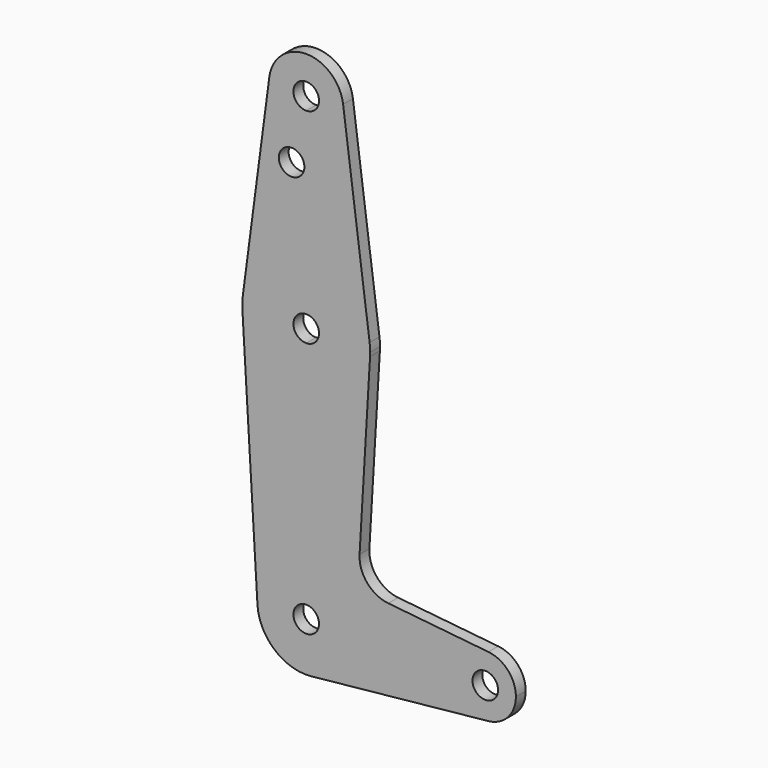
from build123d import *

# Parameters (mm, degrees)
F0_R     = 3.175
F1_DEPTH = 3.048


with BuildPart() as f1:
    # F0 (on Front) → F1 (new body)
    with BuildSketch(Plane.XZ):
        with BuildLine():
            Line((12.1285329959, 0), (3.175, 0))
            ThreePointArc((3.175, 0), (-2.2450640303, -2.2450640303), (0, 3.175))
            Line((0, 3.175), (0, 12.1285329959))
            ThreePointArc((0, 12.1285329959), (-8.8255371973, 8.3193272451), (-12.1074052539, -0.7155771445))
            ThreePointArc((-12.1074052539, -0.7155771445), (-7.858618829, -9.2381503956), (1.2349249899, -12.0654992811))
            ThreePointArc((1.2349249899, -12.0654992811), (9.002198096, -8.1278374782), (12.1285329959, 0))
        make_face()
        with BuildLine():
            ThreePointArc((0, 12.1285329959), (8.5761679272, 8.5761679272), (12.1285329959, 0))
            Line((12.1285329959, 0), (36.8473577956, 0))
            ThreePointArc((36.8473577956, 0), (39.3551513268, 5.6429323481), (45.2240996253, 7.5631301892))
            Line((45.2240996253, 7.5631301892), (20.3690705941, 10.1070859559))
            ThreePointArc((20.3690705941, 10.1070859559), (15.1229915635, 12.8646775774), (13.2422076318, 18.4850253022))
            Line((13.2422076318, 18.4850253022), (15.8473459627, 62.563383249))
            ThreePointArc((15.8473459627, 62.563383249), (10.8891421627, 51.9482811685), (0, 47.625))
            Line((0, 47.625), (0, 12.1285329959))
        make_face()
        with BuildLine():
            Line((36.8473577956, 0), (12.1285329959, 0))
            ThreePointArc((12.1285329959, 0), (9.002198096, -8.1278374782), (1.2349249899, -12.0654992811))
            Line((1.2349249899, -12.0654992811), (45.2240996253, -7.5631301892))
            ThreePointArc((45.2240996253, -7.5631301892), (39.3551513268, -5.6429323481), (36.8473577956, 0))
        make_face()
        with BuildLine():
            ThreePointArc((-12.1074052539, -0.7155771445), (-8.8255371973, 8.3193272451), (0, 12.1285329959))
            Line((0, 12.1285329959), (0, 47.625))
            ThreePointArc((0, 47.625), (-10.8891421627, 51.9482811685), (-15.8473459627, 62.563383249))
            Line((-15.8473459627, 62.563383249), (-12.1074052539, -0.7155771445))
        make_face()
        with BuildLine():
            ThreePointArc((45.2240996253, 7.5631301892), (39.3551513268, 5.6429323481), (36.8473577956, 0))
            ThreePointArc((36.8473577956, 0), (39.3551513268, -5.6429323481), (45.2240996253, -7.5631301892))
            ThreePointArc((45.2240996253, -7.5631301892), (50.0929323481, -5.0948486732), (52.0526422044, 0))
            ThreePointArc((52.0526422044, 0), (50.0929323481, 5.0948486732), (45.2240996253, 7.5631301892))
        make_face()
        with BuildLine():
            ThreePointArc((47.625, 0), (44.45, -3.175), (41.275, 0))
            ThreePointArc((41.275, 0), (44.45, 3.175), (47.625, 0))
        make_face(mode=Mode.SUBTRACT)
        with BuildLine():
            ThreePointArc((-15.8473459627, 62.563383249), (-10.8891421627, 51.9482811685), (0, 47.625))
            Line((0, 47.625), (0, 60.325))
            ThreePointArc((0, 60.325), (-3.175, 63.5), (0, 66.675))
            Line((0, 66.675), (0, 79.375))
            ThreePointArc((0, 79.375), (-10.4661659349, 75.4362890222), (-15.7388575186, 65.5746057477))
            ThreePointArc((-15.7388575186, 65.5746057477), (-15.8647069883, 64.071574295), (-15.8473459627, 62.563383249))
        make_face()
        with BuildLine():
            Line((0, 60.325), (0, 47.625))
            ThreePointArc((0, 47.625), (10.8891421627, 51.9482811685), (15.8473459627, 62.563383249))
            ThreePointArc((15.8473459627, 62.563383249), (15.8680849846, 63.0314875444), (15.875, 63.5))
            ThreePointArc((15.875, 63.5), (15.8409278154, 64.5395340042), (15.7388575186, 65.5746057477))
            ThreePointArc((15.7388575186, 65.5746057477), (10.4661659349, 75.4362890222), (0, 79.375))
            Line((0, 79.375), (0, 66.675))
            ThreePointArc((0, 66.675), (2.2450640303, 65.7450640303), (3.175, 63.5))
            ThreePointArc((3.175, 63.5), (2.2450640303, 61.2549359697), (0, 60.325))
        make_face()
        with BuildLine():
            Line((-9.1570523114, 115.5070300106), (-15.7388575186, 65.5746057477))
            ThreePointArc((-15.7388575186, 65.5746057477), (-10.4661659349, 75.4362890222), (0, 79.375))
            Line((0, 79.375), (0, 105.0637383927))
            ThreePointArc((0, 105.0637383927), (-6.9446732617, 108.2106616314), (-9.1570523114, 115.5070300106))
        make_face()
        with Locations((-3.6322516389, 98.6820235848)):
            Circle(F0_R, mode=Mode.SUBTRACT)
        with BuildLine():
            Line((0, 105.0637383927), (0, 79.375))
            ThreePointArc((0, 79.375), (10.4661659349, 75.4362890222), (15.7388575186, 65.5746057477))
            Line((15.7388575186, 65.5746057477), (9.1570523114, 115.5070300106))
            ThreePointArc((9.1570523114, 115.5070300106), (9.2164380099, 114.9048131032), (9.2362616073, 114.3))
            ThreePointArc((9.2362616073, 114.3), (6.5310232154, 107.7689767846), (0, 105.0637383927))
        make_face()
        with BuildLine():
            ThreePointArc((9.1570523114, 115.5070300106), (0, 123.5362616073), (-9.1570523114, 115.5070300106))
            ThreePointArc((-9.1570523114, 115.5070300106), (-6.9446732617, 108.2106616314), (0, 105.0637383927))
            ThreePointArc((0, 105.0637383927), (6.5310232154, 107.7689767846), (9.2362616073, 114.3))
            ThreePointArc((9.2362616073, 114.3), (9.2164380099, 114.9048131032), (9.1570523114, 115.5070300106))
        make_face()
        with BuildLine():
            ThreePointArc((3.175, 114.3), (2.2450640303, 112.0549359697), (0, 111.125))
            ThreePointArc((0, 111.125), (-2.2450640303, 116.5450640303), (3.175, 114.3))
        make_face(mode=Mode.SUBTRACT)
        with BuildLine():
            ThreePointArc((0, 3.175), (2.2450640303, 2.2450640303), (3.175, 0))
            Line((3.175, 0), (12.1285329959, 0))
            ThreePointArc((12.1285329959, 0), (8.5761679272, 8.5761679272), (0, 12.1285329959))
            Line((0, 12.1285329959), (0, 3.175))
        make_face()
    extrude(amount=F1_DEPTH)


solid = f1.part
